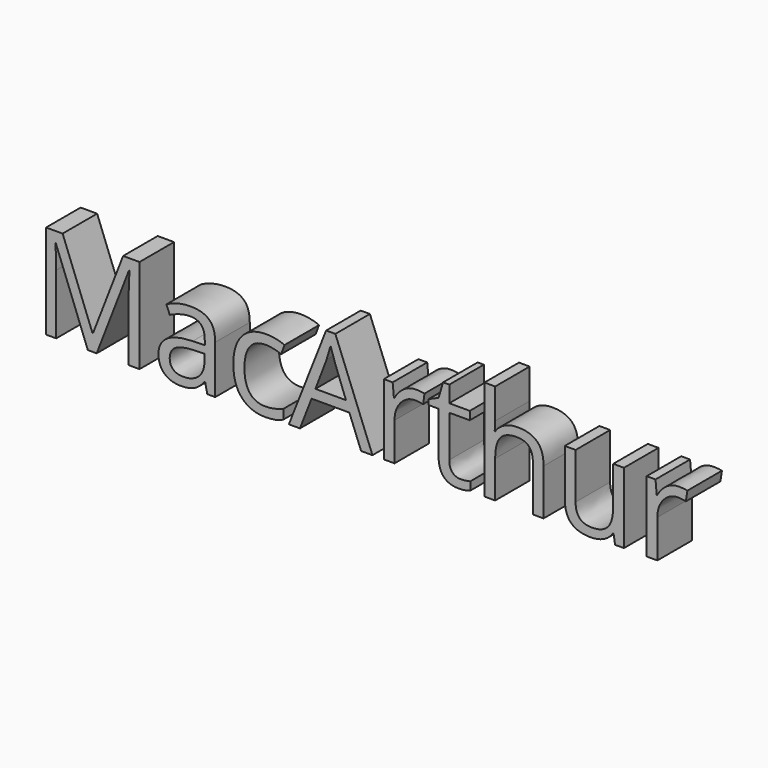
from build123d import *

# Parameters (mm, degrees)
F0_TEXT_SIZE = 77.7392273044
F1_DEPTH     = 25.4


# Not quite as in the source:
# - Text() gives the source's letters only with a copy of the font that has no kerning and outlines rounded to 1/6400 em; it was checked with that copy


with BuildPart() as f1:
    # F0 (on Front) → F1 (new body)
    with BuildSketch(Plane.XZ):
        with Locations((-205.6980058551, -6.5967328846)):
            Text('MacArthur', F0_TEXT_SIZE, font='Open Sans', text_align=(TextAlign.LEFT, TextAlign.BOTTOM))
    extrude(amount=F1_DEPTH)


solid = f1.part
